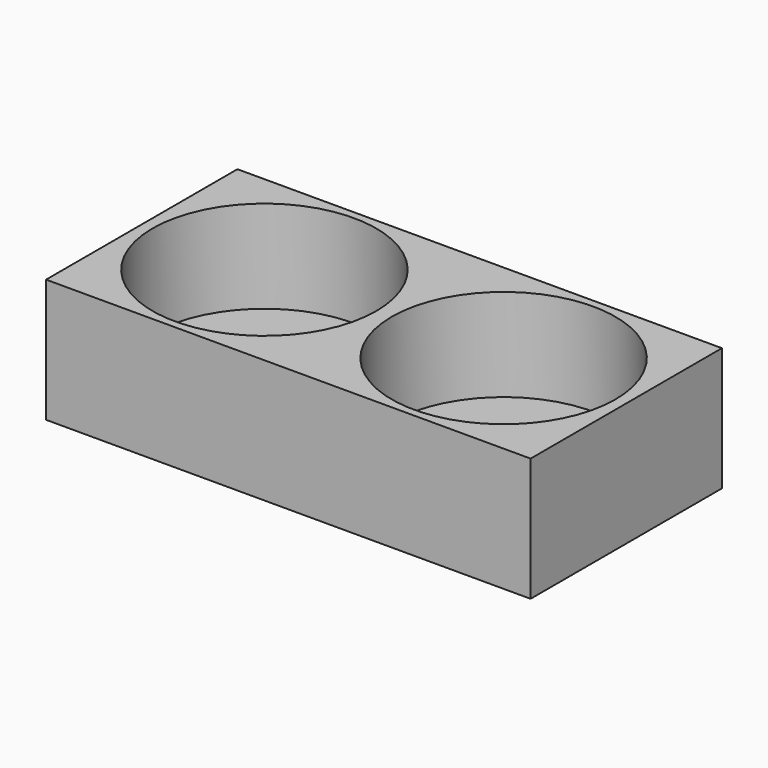
from build123d import *

# Parameters (mm, degrees)
F2_W     = 31.4
F2_H     = 15.5
F3_DEPTH = 8
F4_R     = 7.25
F5_DEPTH = 6


# Not quite as in the source:
# - a feature names something its author has since deleted; it is built from what else it names


with BuildPart() as f3:
    # F2 (on Top) → F3 (new body)
    with BuildSketch(Plane.XY):
        Rectangle(F2_W, F2_H)
    extrude(amount=F3_DEPTH)

    # F4 (on face) → F5 (cut)
    with BuildSketch(Plane.XY.offset(8)):
        with Locations((-7.75, 0)):
            Circle(F4_R)
        with Locations((7.75, 0)):
            Circle(F4_R)
    extrude(amount=-F5_DEPTH, mode=Mode.SUBTRACT)


solid = f3.part
